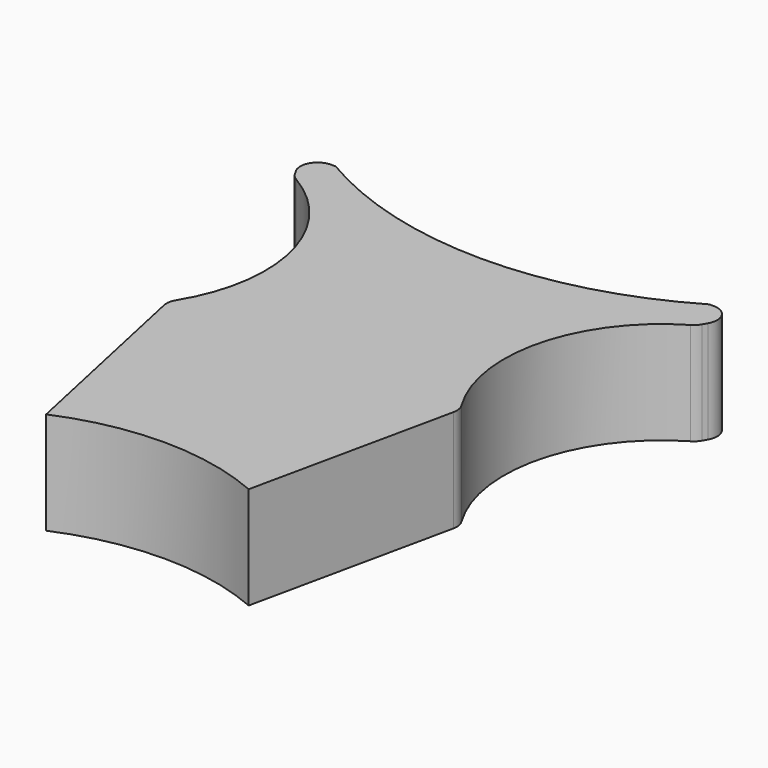
from build123d import *

# Parameters (mm, degrees)
F1_DEPTH = 3
F2_R     = 1


# Not quite as in the source:
# - a feature names something its author has since deleted; it is built from what else it names


with BuildPart() as f1:
    # F0 (on Top) → F1 (new body, symmetric)
    with BuildSketch(Plane.XY):
        with BuildLine():
            Line((-12.9470113486, 10.248668018), (-11.7864680784, 8.248668018))
            ThreePointArc((-11.7864680784, 8.248668018), (-7.2595115052, 2.3329471863), (-8.5698451786, -5))
            Line((-8.5698451786, -5), (-5.9368219527, -17.2248722292))
            ThreePointArc((-5.9368219527, -17.2248722292), (0, -16), (5.9368219527, -17.2248722292))
            Line((5.9368219527, -17.2248722292), (8.5698451786, -5))
            ThreePointArc((8.5698451786, -5), (7.2595115052, 2.3329471863), (11.7864680784, 8.248668018))
            Line((11.7864680784, 8.248668018), (12.9470113486, 10.248668018))
            Line((12.9470113486, 10.248668018), (10.9470113486, 10.248668018))
            ThreePointArc((10.9470113486, 10.248668018), (0, 7.2662124228), (-10.9470113486, 10.248668018))
            Line((-10.9470113486, 10.248668018), (-12.9470113486, 10.248668018))
        make_face()
    extrude(amount=F1_DEPTH, both=True)

    # F2
    f2_edges = [f1.edges().sort_by_distance(p)[0] for p in [
        (-12.947011, 10.248668, 0),
        (12.947011, 10.248668, 0),
        (-8.569845, -5, 0),
        (8.569845, -5, 0),
        (11.786468, 8.248668, 0),
        (-11.786468, 8.248668, 0),
    ]]
    fillet(f2_edges, radius=F2_R)


solid = f1.part
